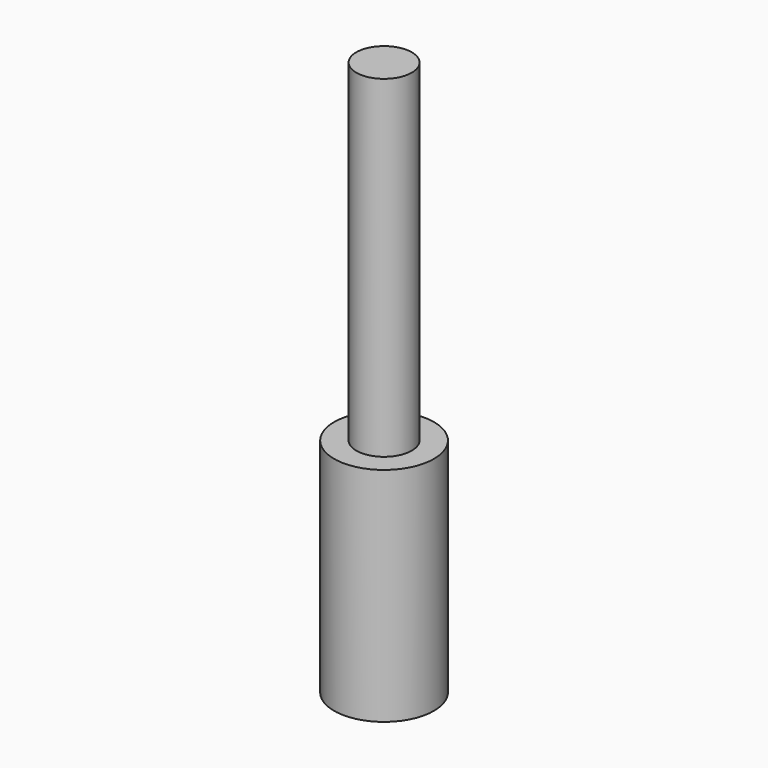
from build123d import *

# Parameters (mm, degrees)
F2_R     = 11.43
F2_R_2   = 6.35
F3_DEPTH = 50.8
F4_DEPTH = 127


# Not quite as in the source:
# - a variable given as a bare number and used for a length is read in inches; the dataset says mm whatever the document's units were


with BuildPart() as f3:
    # F2 (on Top) → F3 (new body)
    with BuildSketch(Plane.XY):
        Circle(F2_R)
        Circle(F2_R_2, mode=Mode.SUBTRACT)
    extrude(amount=F3_DEPTH)

    # F2 (on Top) → F4 (join)
    with BuildSketch(Plane.XY):
        Circle(F2_R_2)
    extrude(amount=F4_DEPTH)


solid = f3.part
